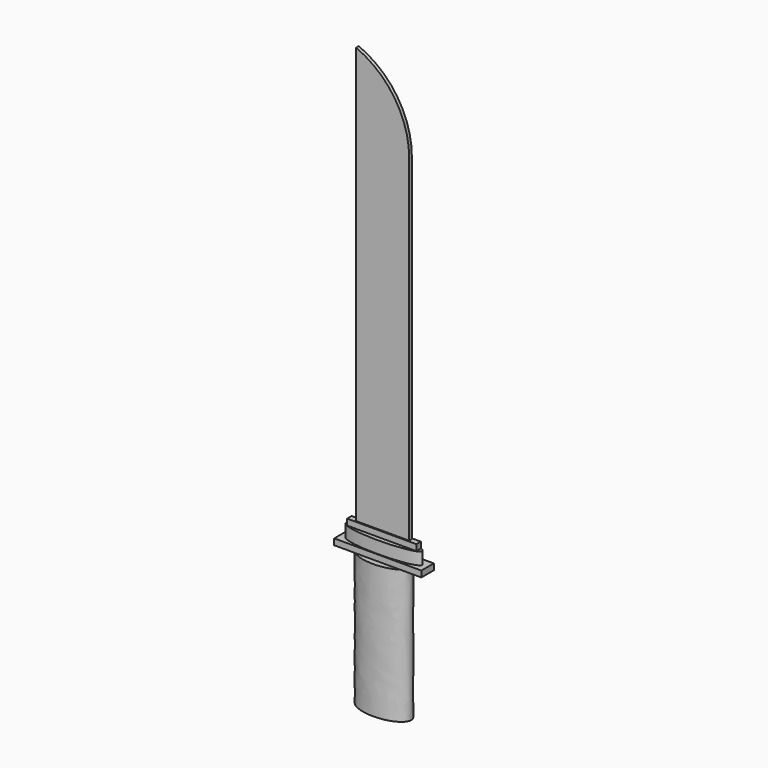
from build123d import *

# Parameters (mm, degrees)
F0_W        = 217.7935391665
F0_H        = 13.5906832293
F1_DEPTH    = 1710
F2_T1_DEPTH = 1658.3004497915
F3_W        = 284.022539854
F3_H        = 23.1398101896
F4_DEPTH    = 25
F7_DEPTH    = 50
F9_W        = 357.4613034725
F9_H        = 63.879750669
F10_DEPTH   = 25
F13_DEPTH   = 550


# Not quite as in the source:
# - a fillet or chamfer that OpenCascade refuses, or shapes differently, is made with other operations: its cross-section is extruded or revolved along the edge and cut away or added


with BuildPart() as f1:
    # F0 (on Top) → F1 (new body)
    with BuildSketch(Plane.XY):
        Rectangle(F0_W, F0_H)
    extrude(amount=F1_DEPTH)

    # F2: fillet of radius 357.3036072312 on 1 edges, made by hand

    # F2_s2 → F2_t1 (cut)
    with BuildSketch(Plane.XZ.offset(-829.1502248957)):
        with BuildLine():
            ThreePointArc((108.8967695832, 1381.0580466876), (49.513720811, 1578.3122192364), (-108.8967695832, 1710))
            Line((-108.8967695832, 1710), (108.8967695832, 1710))
            Line((108.8967695832, 1710), (108.8967695832, 1381.0580466876))
        make_face()
    extrude(amount=F2_T1_DEPTH, mode=Mode.SUBTRACT)

    # F3 (on Top) → F4 (join)
    with BuildSketch(Plane.XY):
        Rectangle(F3_W, F3_H)
    extrude(amount=-F4_DEPTH)

    # F6 (on offset) → F7 (join)
    with BuildSketch(Plane.XY.offset(-25)):
        with BuildLine():
            add(Edge.make_bspline(
                [(157.1267843246, 0), (157.1267843246, 51.8759819398), (-78.5633921623, 25.9379909699), (-314.2535686493, 0), (-78.5633921623, -25.9379909699), (157.1267843246, -51.8759819398), (157.1267843246, 0)],
                knots=[0, 0, 0, 2.0943951024, 2.0943951024, 4.1887902048, 4.1887902048, 6.2831853072, 6.2831853072, 6.2831853072], degree=2, weights=[1, 0.5, 1, 0.5, 1, 0.5, 1]))
        make_face()
    extrude(amount=-F7_DEPTH)

    # F9 (on offset) → F10 (join)
    with BuildSketch(Plane.XY.offset(-75)):
        Rectangle(F9_W, F9_H)
    extrude(amount=-F10_DEPTH)

    # F12 (on offset) → F13 (join)
    with BuildSketch(Plane.XY.offset(-100)):
        with BuildLine():
            add(Edge.make_bspline(
                [(111.7473468184, 0), (111.7473468184, 96.4192818942), (-55.8736734092, 48.2096409471), (-223.4946936369, 0), (-55.8736734092, -48.2096409471), (111.7473468184, -96.4192818942), (111.7473468184, 0)],
                knots=[0, 0, 0, 2.0943951024, 2.0943951024, 4.1887902048, 4.1887902048, 6.2831853072, 6.2831853072, 6.2831853072], degree=2, weights=[1, 0.5, 1, 0.5, 1, 0.5, 1]))
        make_face()
    extrude(amount=-F13_DEPTH)


solid = f1.part
